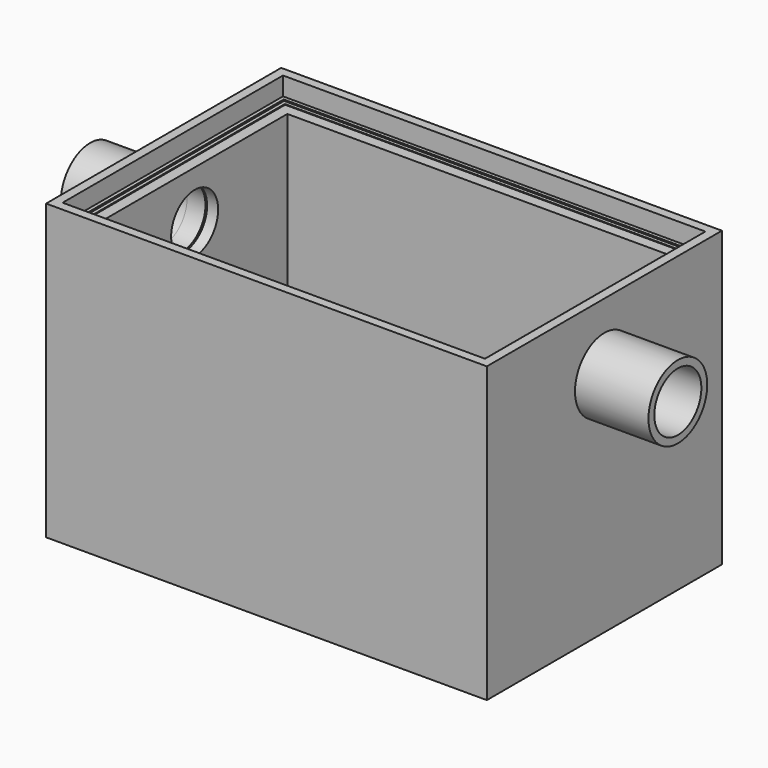
from build123d import *

# Parameters (mm, degrees)
F0_W          = 152.4
F0_H          = 101.6
F1_DEPTH      = 101.6
F2_R          = 12.7
F2_R_2        = 10.16
F3_DEPTH      = 25.4
F3_DEPTH_BACK = 177.8
F4_R          = 10.16
F5_DEPTH      = 152.4
F6_W          = 139.7
F6_H          = 88.9
F7_DEPTH      = 95.25
F8_W          = 146.05
F8_H          = 95.25
F9_DEPTH      = 6.35
F10_W         = 6.35
F10_H         = 82.55
F11_DEPTH     = 3.175
F12_W         = 143.51
F12_H         = 92.71
F12_W_2       = 142.24
F12_H_2       = 91.44
F13_DEPTH     = 0.635
F14_R         = 15.24
F14_R_2       = 12.7
F15_DEPTH     = 3.175
F16_R         = 15.24
F16_R_2       = 12.7
F17_DEPTH     = 3.175
F18_W         = 6.35
F18_H         = 82.55
F19_DEPTH     = 3.175
F21_DEPTH     = 82.042
F22_W         = 5.334
F22_H         = 3.175
F23_DEPTH     = 41.021
F24_T         = 3.81
F24_T3_DEPTH  = 48.641
F24_T5_DEPTH  = 12.954
F24_T7_DEPTH  = 12.954
F25_W         = 138.684
F25_H         = 87.884
F25_W_2       = 131.064
F25_H_2       = 80.264
F26_DEPTH     = 6.985
F27_R         = 10.1600221016
F28_DEPTH     = 152.4


# Not quite as in the source:
# - a shell that OpenCascade refuses in one call is made with other operations: the cavity is built on its own and cut out


with BuildPart() as f1:
    # F0 (on Front) → F1 (new body)
    with BuildSketch(Plane.XZ):
        Rectangle(F0_W, F0_H)
    extrude(amount=F1_DEPTH)

    # F2 (on face) → F3 (join, two sides)
    with BuildSketch(Plane(origin=(-76.2, 0, 0), x_dir=(0, -1, 0), z_dir=(-1, 0, 0))) as f3_sk:
        with Locations((50.8, 27.6547968388)):
            Circle(F2_R)
        with Locations((50.8, 27.6547968388)):
            Circle(F2_R_2, mode=Mode.SUBTRACT)
    extrude(amount=F3_DEPTH)
    extrude(f3_sk.sketch, amount=-F3_DEPTH_BACK)

    # F4 (on face) → F5 (cut)
    with BuildSketch(Plane(origin=(-76.2, 0, 0), x_dir=(0, -1, 0), z_dir=(-1, 0, 0))):
        with Locations((50.8, 27.6547968388)):
            Circle(F4_R)
    extrude(amount=-F5_DEPTH, mode=Mode.SUBTRACT)

    # F6 (on face) → F7 (cut)
    with BuildSketch(Plane.XY.offset(50.8)):
        with Locations((0, -50.8)):
            Rectangle(F6_W, F6_H)
    extrude(amount=-F7_DEPTH, mode=Mode.SUBTRACT)

    # F8 (on face) → F9 (cut)
    with BuildSketch(Plane.XY.offset(50.8)):
        with Locations((0, -50.8)):
            Rectangle(F8_W, F8_H)
    extrude(amount=-F9_DEPTH, mode=Mode.SUBTRACT)

    # F10 (on face) → F11 (cut)
    with BuildSketch(Plane.XZ.offset(6.35)):
        with Locations((-53.975, -3.175)):
            Rectangle(F10_W, F10_H)
        with Locations((53.975, -3.175)):
            Rectangle(F10_W, F10_H)
    extrude(amount=-F11_DEPTH, mode=Mode.SUBTRACT)

    # F12 (on face) → F13 (cut)
    with BuildSketch(Plane.XY.offset(44.45)):
        with Locations((0, -50.8)):
            Rectangle(F12_W, F12_H)
        with Locations((0, -50.8)):
            Rectangle(F12_W_2, F12_H_2, mode=Mode.SUBTRACT)
    extrude(amount=-F13_DEPTH, mode=Mode.SUBTRACT)

    # F14 (on face) → F15 (cut)
    with BuildSketch(Plane.YZ.offset(-69.85)):
        with Locations((-50.8, 27.6547968388)):
            Circle(F14_R)
        with Locations((-50.8, 27.6547968388)):
            Circle(F14_R_2, mode=Mode.SUBTRACT)
    extrude(amount=-F15_DEPTH, mode=Mode.SUBTRACT)

    # F16 (on face) → F17 (cut)
    with BuildSketch(Plane(origin=(69.85, 0, 0), x_dir=(0, -1, 0), z_dir=(-1, 0, 0))):
        with Locations((50.8, 27.6547968388)):
            Circle(F16_R)
        with Locations((50.8, 27.6547968388)):
            Circle(F16_R_2, mode=Mode.SUBTRACT)
    extrude(amount=-F17_DEPTH, mode=Mode.SUBTRACT)

    # F18 (on face) → F19 (cut)
    with BuildSketch(Plane(origin=(0, -95.25, 0), x_dir=(-1, 0, 0), z_dir=(0, 1, 0))):
        with Locations((53.975, -3.175)):
            Rectangle(F18_W, F18_H)
        with Locations((-53.975, -3.175)):
            Rectangle(F18_W, F18_H)
    extrude(amount=-F19_DEPTH, mode=Mode.SUBTRACT)


with BuildPart() as f21:
    # F20 (on face) → F21 (new body)
    with BuildSketch(Plane.XY.offset(-44.45)):
        Polygon((51.308, -97.917), (56.642, -97.917), (56.642, -94.742), (69.342, -94.742), (69.342, -6.858), (56.642, -6.858), (56.642, -3.683), (51.308, -3.683), (51.308, -6.858), (-51.308, -6.858), (-51.308, -3.683), (-56.642, -3.683), (-56.642, -6.858), (-69.342, -6.858), (-69.342, -94.742), (-56.642, -94.742), (-56.642, -97.917), (-51.308, -97.917), (-51.308, -94.742), (51.308, -94.742), align=None)
    extrude(amount=F21_DEPTH)

    # F22 (on face) → F23 (cut)
    with BuildSketch(Plane.XY.offset(37.592)):
        with Locations((53.975, -5.2705)):
            Rectangle(F22_W, F22_H)
        with Locations((53.975, -96.3295)):
            Rectangle(F22_W, F22_H)
        with Locations((-53.975, -96.3295)):
            Rectangle(F22_W, F22_H)
        with Locations((-53.975, -5.2705)):
            Rectangle(F22_W, F22_H)
    extrude(amount=-F23_DEPTH, mode=Mode.SUBTRACT)

    # F24: shell of thickness 3.81, made by hand


with BuildPart() as f24_core1:
    # F24_t2: copy of F21
    add(f21.part)

    # the walls: a layer under each face that stays
    f24_faces = [f24_core1.faces().sort_by_distance(p)[0] for p in [
        (53.975, -97.917, -23.9395),
        (51.308, -96.3295, -23.9395),
        (0, -94.742, -3.429),
        (69.342, -50.8, -3.429),
        (0, -6.858, -3.429),
        (56.642, -5.2705, -23.9395),
        (53.975, -3.683, -23.9395),
        (53.975, -5.2705, -3.429),
        (51.308, -5.2705, -23.9395),
        (-51.308, -5.2705, -23.9395),
        (-53.975, -3.683, -23.9395),
        (-53.975, -5.2705, -3.429),
        (-56.642, -5.2705, -23.9395),
        (-69.342, -50.8, -3.429),
        (-56.642, -96.3295, -23.9395),
        (-53.975, -97.917, -23.9395),
        (-53.975, -96.3295, -3.429),
        (-51.308, -96.3295, -23.9395),
        (53.975, -96.3295, -3.429),
        (56.642, -96.3295, -23.9395),
        (0, -50.8, -44.45),
    ]]
    thicken(f24_faces, amount=-F24_T, mode=Mode.SUBTRACT)

    # F24_s4 → F24_t3 (cut)
    with BuildSketch(Plane.XY.offset(-48.26)):
        Polygon((51.2699, -94.7801), (55.118, -94.742), (55.118, -90.932), (51.308, -90.932), align=None)
        Polygon((56.6801, -94.7801), (56.642, -90.932), (52.832, -90.932), (52.832, -94.742), align=None)
        Polygon((-51.2699, -94.7801), (-51.308, -90.932), (-55.118, -90.932), (-55.118, -94.742), align=None)
        Polygon((-56.6801, -94.7801), (-56.642, -90.932), (-52.832, -90.932), (-52.832, -94.742), align=None)
        Polygon((-56.6801, -6.8199), (-56.642, -10.668), (-52.832, -10.668), (-52.832, -6.858), align=None)
        Polygon((-51.2699, -6.8199), (-51.308, -10.668), (-55.118, -10.668), (-55.118, -6.858), align=None)
        Polygon((51.2699, -6.8199), (51.308, -10.668), (55.118, -10.668), (55.118, -6.858), align=None)
        Polygon((56.6801, -6.8199), (56.642, -10.668), (52.832, -10.668), (52.832, -6.858), align=None)
    extrude(amount=F24_T3_DEPTH, mode=Mode.SUBTRACT)

    # F24_s6 → F24_t5 (cut)
    with BuildSketch(Plane.YZ.offset(47.498)):
        Polygon((-94.7801, -3.3909), (-90.932, -3.429), (-90.932, -7.239), (-94.742, -7.239), align=None)
        Polygon((-6.8199, -3.3909), (-10.668, -3.429), (-10.668, -7.239), (-6.858, -7.239), align=None)
    extrude(amount=F24_T5_DEPTH, mode=Mode.SUBTRACT)

    # F24_s8 → F24_t7 (cut)
    with BuildSketch(Plane.YZ.offset(-60.452)):
        Polygon((-94.7801, -3.3909), (-90.932, -3.429), (-90.932, -7.239), (-94.742, -7.239), align=None)
        Polygon((-6.8199, -3.3909), (-10.668, -3.429), (-10.668, -7.239), (-6.858, -7.239), align=None)
    extrude(amount=F24_T7_DEPTH, mode=Mode.SUBTRACT)


with BuildPart() as f21_1:
    add(f21.part)

    # what is left inside the walls is the cavity
    f24_cavity = [f24_core1.part.solids().sort_by_distance(p)[0] for p in [
        (0, -64.177333, -40.6019),
    ]]
    add(f24_cavity, mode=Mode.SUBTRACT)

    # F25 (on face) → F26 (join)
    with BuildSketch(Plane.XY.offset(37.592)):
        with Locations((0, -50.8)):
            Rectangle(F25_W, F25_H)
        with Locations((0, -50.8)):
            Rectangle(F25_W_2, F25_H_2, mode=Mode.SUBTRACT)
    extrude(amount=F26_DEPTH)

    # F27 (on face) → F28 (cut)
    with BuildSketch(Plane.YZ.offset(69.342)):
        with Locations((-50.732751833, 27.6044615543)):
            Circle(F27_R)
    extrude(amount=-F28_DEPTH, mode=Mode.SUBTRACT)


solid = Compound([f1.part, f21_1.part])
